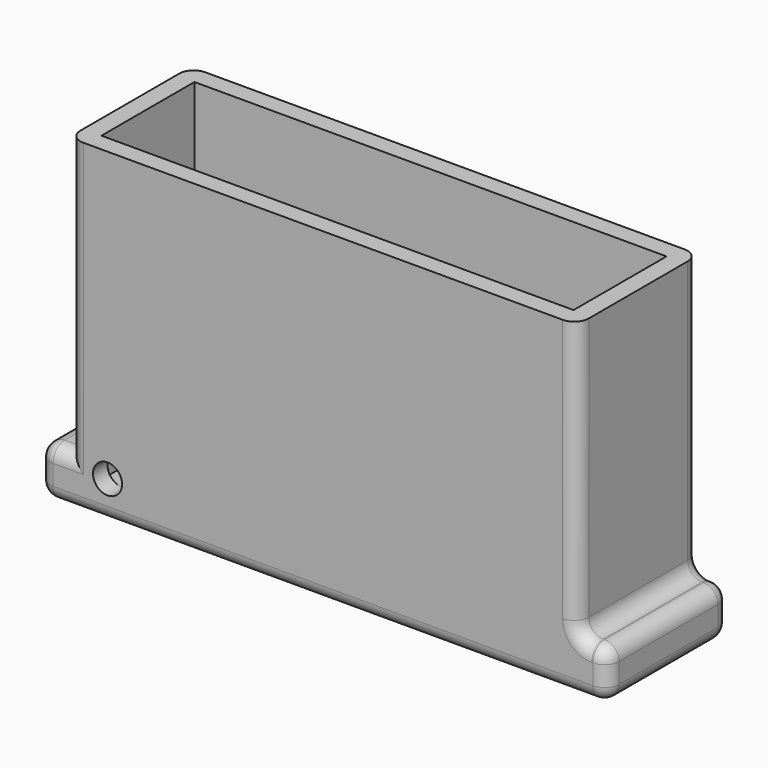
from build123d import *

# Parameters (mm, degrees)
F0_W         = 19.5
F0_H         = 4.8
F1_DEPTH     = 1
F0_W_2       = 21
F0_H_2       = 6.3
F2_DEPTH     = 13.5
F0_W_3       = 1.25
F3_DEPTH     = 2.03371
F4_R         = 0.6
F5_R         = 0.6
F6_DEPTH     = 2
F7_TEXT_SIZE = 3.5643908991
F8_DEPTH     = 0.6


# Not quite as in the source:
# - Text() gives the source's letters only with a copy of the font that has no kerning and outlines rounded to 1/6400 em; it was checked with that copy


with BuildPart() as f1:
    # F0 (on Top) → F1 (new body)
    with BuildSketch(Plane.XY):
        Rectangle(F0_W, F0_H)
    extrude(amount=F1_DEPTH)

    # F0 (on Top) → F2 (join)
    with BuildSketch(Plane.XY):
        Rectangle(F0_W_2, F0_H_2)
        Rectangle(F0_W, F0_H, mode=Mode.SUBTRACT)
    extrude(amount=F2_DEPTH)

    # F0 (on Top) → F3 (join)
    with BuildSketch(Plane.XY):
        with Locations((-11.125, 0)):
            Rectangle(F0_W_3, F0_H_2)
        with Locations((11.125, 0)):
            Rectangle(F0_W_3, F0_H_2)
    extrude(amount=F3_DEPTH)

    # F4
    f4_edges = [f1.edges().sort_by_distance(p)[0] for p in [
        (-11.75, 0, 2.03371),
        (11.75, 0, 2.03371),
        (11.75, -3.15, 1.016855),
        (11.125, 3.15, 2.03371),
        (10.5, 0, 2.03371),
        (11.125, -3.15, 2.03371),
        (-11.125, -3.15, 2.03371),
        (-10.5, -3.15, 7.766855),
        (-11.125, 3.15, 2.03371),
        (-10.5, 3.15, 7.766855),
        (-11.75, 3.15, 1.016855),
        (-11.75, -3.15, 1.016855),
        (0, 3.15, 0),
        (0, -3.15, 0),
        (11.75, 0, 0),
        (-11.75, 0, 0),
        (11.75, 3.15, 1.016855),
        (10.5, 3.15, 7.766855),
        (10.5, -3.15, 7.766855),
    ]]
    fillet(f4_edges, radius=F4_R)

    # F5 (on face) → F6 (cut)
    with BuildSketch(Plane.XZ.offset(3.15)):
        with Locations((-8.9, 1.6001462936)):
            Circle(F5_R)
    extrude(amount=-F6_DEPTH, mode=Mode.SUBTRACT)

    # F7 (on face) → F8 (cut)
    with BuildSketch(Plane(origin=(0, 0, 0), x_dir=(1, 0, 0), z_dir=(0, 0, -1))):
        Polygon((-9.3128626441, 0.9369742875), (-9.9817580472, 0.9369742875), (-8.9243204465, -0.2877279387), (-8.0446758379, 0.9363311961), (-8.7135712409, 0.9363311961), (-8.7135712409, 2.5029374722), (-9.3128626441, 2.5029374722), align=None)
        with Locations((-7.5, -1.3441120759)):
            Text('MDI e-Fuse', F7_TEXT_SIZE, font='Open Sans', font_style=FontStyle.BOLDITALIC, text_align=(TextAlign.LEFT, TextAlign.BOTTOM))
    extrude(amount=-F8_DEPTH, mode=Mode.SUBTRACT)


solid = f1.part
